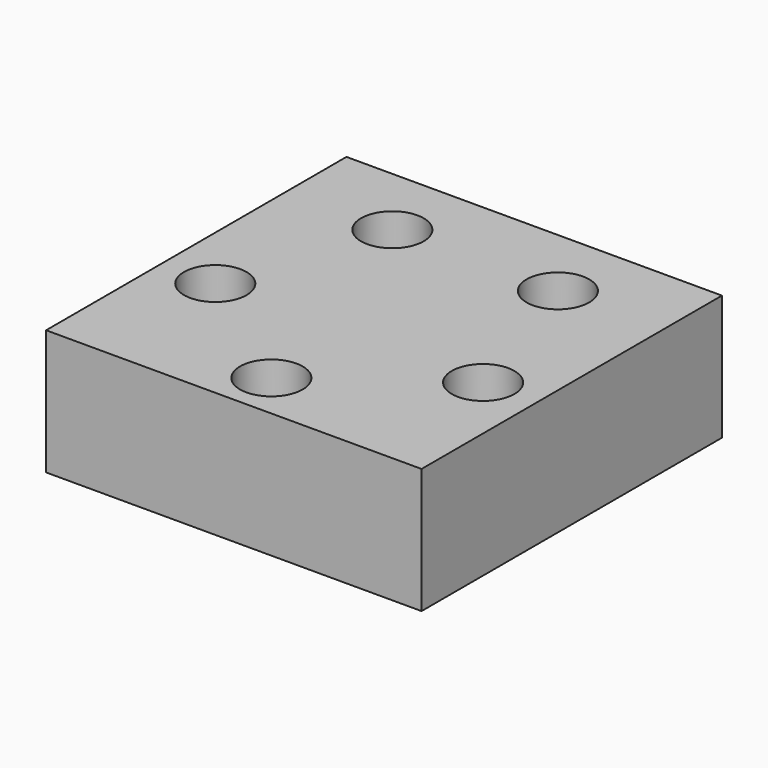
from build123d import *

# Parameters (mm, degrees)
F0_W            = 76.2
F0_H            = 76.2
F1_DEPTH        = 25.4
F2_R            = 6.35
F3_DEPTH        = 12.7
F3_COPIES_COUNT = 5


# Not quite as in the source:
# - a pattern or mirror of a feature is missing from the dataset's text; its kind, count and spacing are read off the source's solid


with BuildPart() as f1:
    # F0 (on Top) → F1 (new body)
    with BuildSketch(Plane.XY):
        Rectangle(F0_W, F0_H)
    extrude(amount=F1_DEPTH)

    # F2 (on face) → F3 (cut)
    with BuildSketch(Plane.XY.offset(25.4)):
        with Locations((0, -28.575)):
            Circle(F2_R)
    f3 = extrude(amount=-F3_DEPTH, mode=Mode.SUBTRACT)

    # F3_copies: F3 ×5 about axis
    f3_copies_axis = Axis((0, 0, 0), (0, 0, 1))
    for i in range(1, F3_COPIES_COUNT):
        add(f3.rotate(f3_copies_axis, i * 360 / F3_COPIES_COUNT), mode=Mode.SUBTRACT)


solid = f1.part
